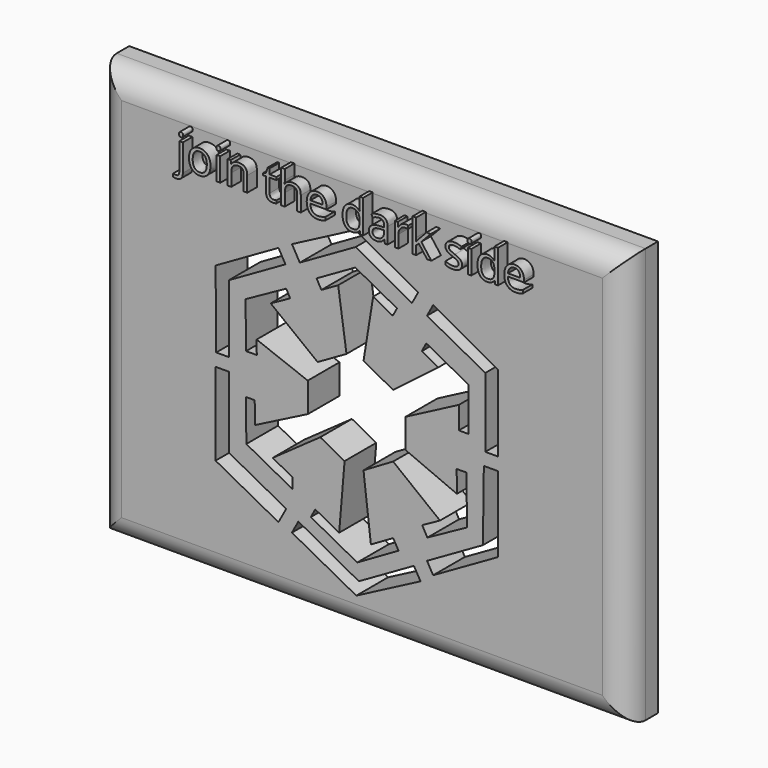
from build123d import *

# Parameters (mm, degrees)
F0_W         = 111.8375621736
F0_H         = 87.8142006695
F1_DEPTH     = 8.382
F2_TEXT_SIZE = 9.2302500788
F3_DEPTH     = 10.922
F4_T1_DEPTH  = 113.2142006695
F4_T3_DEPTH  = 137.2375621736
F4_T8_DEPTH  = 137.2375621736
F4_T13_DEPTH = 137.2375621736
F4_T18_DEPTH = 137.2375621736
F4_T24_DEPTH = 137.2375621736
F4_T30_DEPTH = 137.2375621736
F4_T36_DEPTH = 137.2375621736


# Not quite as in the source:
# - a fillet or chamfer that OpenCascade refuses, or shapes differently, is made with other operations: its cross-section is extruded or revolved along the edge and cut away or added
# - Text() gives the source's letters only with a copy of the font that has no kerning and outlines rounded to 1/6400 em; it was checked with that copy


with BuildPart() as f1:
    # F0 (on Front) → F1 (new body)
    with BuildSketch(Plane.XZ):
        with Locations((-0.3393124789, 11.3330539316)):
            Rectangle(F0_W, F0_H)
        Polygon((-15.1333585382, -18.5679033264), (-13.7761067599, -16.0395860462), (-0.9907946949, -23.0189921312), (10.6654674139, -16.3582723253), (12.053269842, -18.7869270846), (-1.524074073, -25.8736420821), align=None, mode=Mode.SUBTRACT)
        Polygon((-31.2846563756, -10.4162943366), (-31.2846563756, 7.0577096194), (-28.4908089383, 7.0577096194), (-28.4908089383, -8.0077862367), (-16.3548849523, -14.5225953311), (-17.9835874587, -17.5565767613), align=None, mode=Mode.SUBTRACT)
        Polygon((-3.5967177246, 18.4586253017), (-5.3611448966, 30.6738931686), (-8.8983522968, 28.6526322216), (-9.93403964, 30.465085453), (-1.730497677, 35.1528227329), (7.0907307068, 30.4174091818), (6.1926901896, 28.744520338), (2.0447660356, 30.9712097959), (0, 18.3228999376), (6.2645609987, 14.9599570736), (15.811983496, 22.2589317709), (12.3139993148, 24.1367203251), (13.2731856425, 25.923512876), (22.1834440337, 21.1403062189), (22.1834440337, 11.9438162073), (20.1551914215, 11.9438162073), (20.1551914215, 16.6941974312), (8.9172926343, 10.828559323), (8.9172926343, 4.6146563254), (19.7480153292, 0), (19.7092366577, 4.6146563254), (21.7894479132, 4.6321371135), (21.8751583093, -5.5673876662), (13.5046578944, -10.1793892682), (12.4170504519, -8.2054483779), (16.1736440316, -6.1356299981), (6.2645609987, 1.6287022736), (0, -2.0358779002), (1.5608392423, -15.3369465843), (6.2645609987, -12.6224430278), (7.4040087099, -14.596890612), (-1.3297636358, -19.6371241381), (-11.1445184925, -14.368365511), (-10.2072720426, -12.6224430278), (-5.1506374822, -15.3369465843), (-4.0038931184, -1.6287022736), (-9.1543911856, 1.136189109), (-19.2051157355, -5.9719081037), (-15.0261538797, -8.2152592268), (-15.0074434469, -10.4417980304), (-24.7802524699, -5.195556774), (-24.8535801977, 3.5304322644), (-23.0054203421, 3.5304322644), (-22.9666024024, -1.0888969661), (-11.7402290925, 4.6146563254), (-11.792446828, 10.828559323), (-22.5982442498, 14.9599570736), (-22.5740695166, 12.083167304), (-24.8535801977, 12.0640117289), (-24.9347163911, 21.719207053), (-16.3548849523, 26.4664106071), (-15.5058869547, 24.9319788877), (-19.6207430553, 22.6552372472), (-9.7043514252, 14.9599570736), align=None, mode=Mode.SUBTRACT)
        Polygon((25.2525789309, -7.7667636555), (25.4484731704, 7.0577096194), (28.4344293177, 7.0577096194), (28.4344293177, -8.957862854), (14.7261843085, -16.791144071), (13.4298710152, -14.5225953311), align=None, mode=Mode.SUBTRACT)
        Polygon((-31.1489310116, 9.7722141072), (-31.2846563756, 25.923512876), (-17.9835874587, 33.5241220891), (-16.5052281319, 30.9369927237), (-28.4908089383, 24.0880908444), (-28.4908089383, 9.7722141072), align=None, mode=Mode.SUBTRACT)
        Polygon((-13.471248212, 32.2441290512), (-15.1333585382, 35.1528227329), (-1.7493583442, 42.1386216856), (11.5608312413, 34.8308363256), (10.2472510189, 32.4383191764), (-1.6756835237, 38.9844503144), align=None, mode=Mode.SUBTRACT)
        Polygon((13.4223313852, 31.0952773238), (14.7261843085, 33.5241220891), (28.4344293177, 25.923512876), (28.4344293177, 9.7722141072), (25.7617571232, 9.7722141072), (25.7617571232, 24.4712243791), align=None, mode=Mode.SUBTRACT)
    extrude(amount=F1_DEPTH)

    # F2 (on Front) → F3 (join)
    with BuildSketch(Plane.XZ):
        with Locations((-37.7245880663, 43.3278977871)):
            Text('join the dark side', F2_TEXT_SIZE, font='Open Sans', text_align=(TextAlign.LEFT, TextAlign.BOTTOM))
    extrude(amount=F3_DEPTH)

    # F4: fillet of radius 5.08 on 4 edges, made by hand

    # F4_s2 → F4_t1 (cut)
    with BuildSketch(Plane.XY.offset(-45.2740464032)):
        with BuildLine():
            ThreePointArc((-56.2580935657, -3.302), (-54.7701960141, -6.8941024484), (-51.1780935657, -8.382))
            Line((-51.1780935657, -8.382), (-56.2580935657, -8.382))
            Line((-56.2580935657, -8.382), (-56.2580935657, -3.302))
        make_face()
        with BuildLine():
            ThreePointArc((55.5794686079, -3.302), (54.0915710563, -6.8941024484), (50.4994686079, -8.382))
            Line((50.4994686079, -8.382), (55.5794686079, -8.382))
            Line((55.5794686079, -8.382), (55.5794686079, -3.302))
        make_face()
    extrude(amount=F4_T1_DEPTH, mode=Mode.SUBTRACT)

    # F4_s4 → F4_t3 (cut)
    with BuildSketch(Plane.YZ.offset(-68.9580935657)):
        with BuildLine():
            ThreePointArc((-8.382, -27.4940464032), (-6.8941024484, -31.0861488516), (-3.302, -32.5740464032))
            Line((-3.302, -32.5740464032), (-8.382, -32.5740464032))
            Line((-8.382, -32.5740464032), (-8.382, -27.4940464032))
        make_face()
    extrude(amount=F4_T3_DEPTH, mode=Mode.SUBTRACT)


with BuildPart() as f4_tool6:
    # F4_s7 → F4_t8 (new body)
    with BuildSketch(Plane.YZ.offset(68.2794686079)):
        with BuildLine():
            ThreePointArc((-3.302, 55.2401542664), (-6.8941024484, 53.7522567148), (-8.382, 50.1601542664))
            Line((-8.382, 50.1601542664), (-8.382, 55.2401542664))
            Line((-8.382, 55.2401542664), (-3.302, 55.2401542664))
        make_face()
    extrude(amount=-F4_T8_DEPTH)

    split(bisect_by=Plane.XY.offset(50.3414456204), keep=Keep.TOP)


with BuildPart() as f1_1:
    add(f1.part)

    # F4_t5: cut F4_tool6
    add(f4_tool6.part, mode=Mode.SUBTRACT)


with BuildPart() as f4_tool11:
    # F4_s12 → F4_t13 (new body)
    with BuildSketch(Plane.YZ.offset(68.2794686079)):
        with BuildLine():
            ThreePointArc((-3.302, 55.2401542664), (-6.8941024484, 53.7522567148), (-8.382, 50.1601542664))
            Line((-8.382, 50.1601542664), (-8.382, 55.2401542664))
            Line((-8.382, 55.2401542664), (-3.302, 55.2401542664))
        make_face()
    extrude(amount=-F4_T13_DEPTH)

    split(bisect_by=Plane.YZ.offset(30.4869600158), keep=Keep.TOP)


with BuildPart() as f1_2:
    add(f1_1.part)

    # F4_t10: cut F4_tool11
    add(f4_tool11.part, mode=Mode.SUBTRACT)


with BuildPart() as f4_tool16:
    # F4_s17 → F4_t18 (new body)
    with BuildSketch(Plane.YZ.offset(68.2794686079)):
        with BuildLine():
            ThreePointArc((-3.302, 55.2401542664), (-6.8941024484, 53.7522567148), (-8.382, 50.1601542664))
            Line((-8.382, 50.1601542664), (-8.382, 55.2401542664))
            Line((-8.382, 55.2401542664), (-3.302, 55.2401542664))
        make_face()
    extrude(amount=-F4_T18_DEPTH)

    split(bisect_by=Plane.YZ.offset(13.1759144384), keep=Keep.TOP)

    split(bisect_by=Plane.YZ.offset(29.7384444235), keep=Keep.BOTTOM)


with BuildPart() as f1_3:
    add(f1_2.part)

    # F4_t15: cut F4_tool16
    add(f4_tool16.part, mode=Mode.SUBTRACT)


with BuildPart() as f4_tool22:
    # F4_s23 → F4_t24 (new body)
    with BuildSketch(Plane.YZ.offset(68.2794686079)):
        with BuildLine():
            ThreePointArc((-3.302, 55.2401542664), (-6.8941024484, 53.7522567148), (-8.382, 50.1601542664))
            Line((-8.382, 50.1601542664), (-8.382, 55.2401542664))
            Line((-8.382, 55.2401542664), (-3.302, 55.2401542664))
        make_face()
    extrude(amount=-F4_T24_DEPTH)

    split(bisect_by=Plane.YZ.offset(1.9481805535), keep=Keep.TOP)

    split(bisect_by=Plane.YZ.offset(12.4360522055), keep=Keep.BOTTOM)


with BuildPart() as f1_4:
    add(f1_3.part)

    # F4_t21: cut F4_tool22
    add(f4_tool22.part, mode=Mode.SUBTRACT)


with BuildPart() as f4_tool28:
    # F4_s29 → F4_t30 (new body)
    with BuildSketch(Plane.YZ.offset(68.2794686079)):
        with BuildLine():
            ThreePointArc((-3.302, 55.2401542664), (-6.8941024484, 53.7522567148), (-8.382, 50.1601542664))
            Line((-8.382, 50.1601542664), (-8.382, 55.2401542664))
            Line((-8.382, 55.2401542664), (-3.302, 55.2401542664))
        make_face()
    extrude(amount=-F4_T30_DEPTH)

    split(bisect_by=Plane.YZ.offset(-14.6157916582), keep=Keep.TOP)

    split(bisect_by=Plane.YZ.offset(1.1996649612), keep=Keep.BOTTOM)


with BuildPart() as f1_5:
    add(f1_4.part)

    # F4_t27: cut F4_tool28
    add(f4_tool28.part, mode=Mode.SUBTRACT)


with BuildPart() as f4_tool34:
    # F4_s35 → F4_t36 (new body)
    with BuildSketch(Plane.YZ.offset(68.2794686079)):
        with BuildLine():
            ThreePointArc((-3.302, 55.2401542664), (-6.8941024484, 53.7522567148), (-8.382, 50.1601542664))
            Line((-8.382, 50.1601542664), (-8.382, 55.2401542664))
            Line((-8.382, 55.2401542664), (-3.302, 55.2401542664))
        make_face()
    extrude(amount=-F4_T36_DEPTH)

    split(bisect_by=Plane.YZ.offset(-15.3643072505), keep=Keep.BOTTOM)


with BuildPart() as f1_6:
    add(f1_5.part)

    # F4_t33: cut F4_tool34
    add(f4_tool34.part, mode=Mode.SUBTRACT)


solid = f1_6.part
